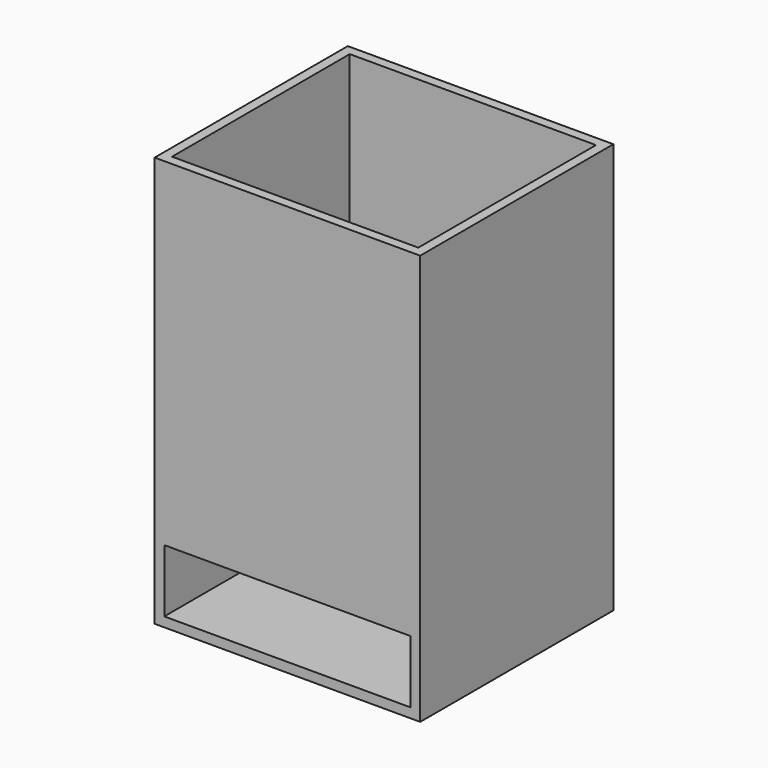
from build123d import *

# Parameters (mm, degrees)
F0_W        = 69.85
F0_H        = 88.9
F1_DEPTH    = 63.5
F2_T        = -2.54
F0_H_2      = 19.05
F3_DEPTH    = 63.5
F4_T        = 2.54
F4_T3_DEPTH = 91.44
F4_T5_DEPTH = 69.85
F4_T7_DEPTH = 63.5


# Not quite as in the source:
# - a shell that OpenCascade refuses in one call is made with other operations: the cavity is built on its own and cut out


with BuildPart() as f1:
    # F0 (on Front) → F1 (new body)
    with BuildSketch(Plane.XZ):
        with Locations((-9.7199578146, -2.0941891145)):
            Rectangle(F0_W, F0_H)
    extrude(amount=F1_DEPTH)

    # F2
    f2_openings = [f1.faces().sort_by_distance(p)[0] for p in [
        (-9.719958, -31.75, 42.355811),
    ]]
    offset(amount=F2_T, openings=f2_openings)

    # F0 (on Front) → F3 (join)
    with BuildSketch(Plane.XZ):
        with Locations((-9.7199578146, -56.0691891145)):
            Rectangle(F0_W, F0_H_2)
    extrude(amount=F3_DEPTH)

    # F4: shell of thickness 2.54, made by hand


with BuildPart() as f4_core1:
    # F4_t2: copy of F1
    add(f1.part)

    # the walls: a layer under each face that stays
    f4_faces = [f4_core1.faces().sort_by_distance(p)[0] for p in [
        (-44.6449578146, -31.75, -11.6191891145),
        (-9.7199578146, 0, -11.6191891145),
        (25.2050421854, -31.75, -11.6191891145),
        (-9.7199578146, -31.75, -65.5941891145),
        (22.8767088521, -61.3833333333, 42.3558108855),
        (-9.7199578146, -60.96, -0.8241891145),
        (-9.7199578146, -31.75, -44.0041891145),
        (-42.1049578146, -31.75, -0.8241891145),
        (-9.7199578146, -2.54, -0.8241891145),
        (22.6650421854, -31.75, -0.8241891145),
    ]]
    thicken(f4_faces, amount=-F4_T, mode=Mode.SUBTRACT)

    # F4_s4 → F4_t3 (cut)
    with BuildSketch(Plane.XY.offset(-46.5441891145)):
        Polygon((-42.0795578146, -60.9346), (-42.1049578146, -63.5), (-44.6449578146, -63.5), (-44.6449578146, -60.96), align=None)
        Polygon((22.6396421854, -60.9346), (22.6650421854, -63.5), (25.2050421854, -63.5), (25.2050421854, -60.96), align=None)
        Polygon((-42.0795578146, -2.5654), (-44.6449578146, -2.54), (-44.6449578146, 0), (-42.1049578146, 0), align=None)
        Polygon((22.6396421854, -2.5654), (22.6650421854, 0), (25.2050421854, 0), (25.2050421854, -2.54), align=None)
    extrude(amount=F4_T3_DEPTH, mode=Mode.SUBTRACT)

    # F4_s6 → F4_t5 (cut)
    with BuildSketch(Plane.YZ.offset(-44.6449578146)):
        Polygon((-60.9346, -43.9787891145), (-63.5, -44.0041891145), (-63.5, -46.5441891145), (-60.96, -46.5441891145), align=None)
        Polygon((-2.5654, -43.9787891145), (-2.54, -46.5441891145), (0, -46.5441891145), (0, -44.0041891145), align=None)
    extrude(amount=F4_T5_DEPTH, mode=Mode.SUBTRACT)

    # F4_s8 → F4_t7 (cut)
    with BuildSketch(Plane.XZ):
        Polygon((22.6396421854, -43.9787891145), (22.6650421854, -46.5441891145), (25.2050421854, -46.5441891145), (25.2050421854, -44.0041891145), align=None)
        Polygon((-42.0795578146, -43.9787891145), (-42.1049578146, -46.5441891145), (-44.6449578146, -46.5441891145), (-44.6449578146, -44.0041891145), align=None)
    extrude(amount=F4_T7_DEPTH, mode=Mode.SUBTRACT)


with BuildPart() as f1_1:
    add(f1.part)

    # what is left inside the walls is the cavity
    f4_cavity = [f4_core1.part.solids().sort_by_distance(p)[0] for p in [
        (-9.719958, -43.18, -63.028789),
    ]]
    add(f4_cavity, mode=Mode.SUBTRACT)


solid = f1_1.part
